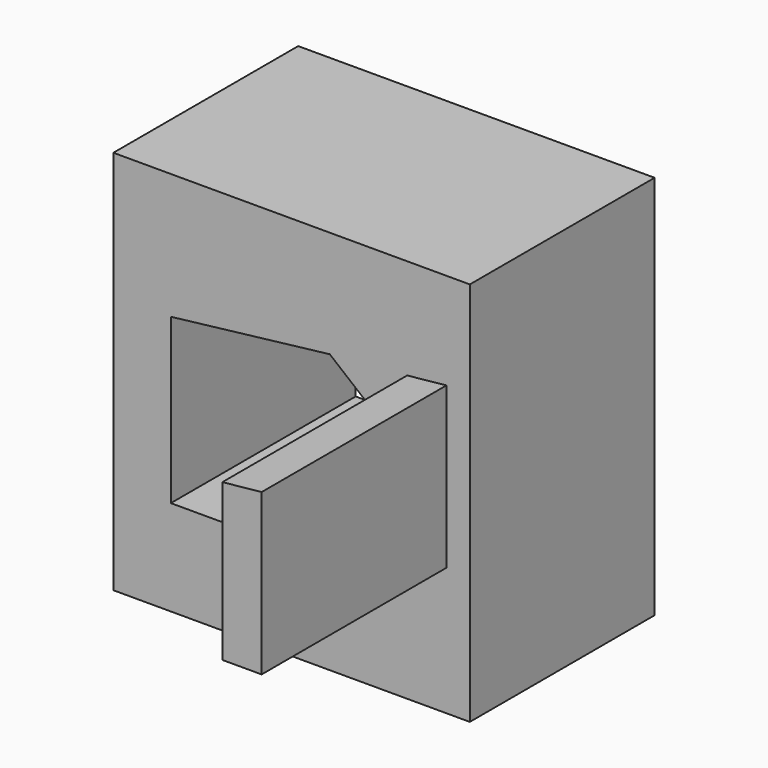
from build123d import *

# Parameters (mm, degrees)
F0_W     = 39.1931459308
F0_H     = 42.3528775573
F1_DEPTH = 25.4
F3_DEPTH = 25.4
F5_DEPTH = 25.4


# Not quite as in the source:
# - ends of sketch curves that miss each other by under 0.0002 mm in the source are joined
# - a feature of the source that left no trace in its solid (it failed there, or was rolled back) is left out


with BuildPart() as f1:
    # F0 (on Front) → F1 (new body)
    with BuildSketch(Plane.XZ):
        with Locations((-19.5965729654, 21.1764387786)):
            Rectangle(F0_W, F0_H)
    extrude(amount=F1_DEPTH)

    # F2 (on face) → F3 (cut)
    with BuildSketch(Plane.XZ.offset(25.4)):
        Polygon((-6.8881497718, 23.612594232), (-15.3977563605, 30.5856615305), (-32.8769646585, 28.529709205), (-32.8769646585, 10.48855111), (-16.7776942253, 10.48855111), (-14.3628085498, 20.764878951), align=None)
        Polygon((-21.8374673277, 17.9171636701), (-14.3628085498, 20.764878951), (-20.9175087512, 15.6267150305), align=None, mode=Mode.SUBTRACT)
        Polygon((-20.9175087512, 15.6267150305), (-14.3628085498, 20.764878951), (-21.8374673277, 17.9171636701), align=None)
    extrude(amount=-F3_DEPTH, mode=Mode.SUBTRACT)

    # F4 (on face) → F5 (join)
    with BuildSketch(Plane.XZ.offset(25.4)):
        Polygon((-6.8881497718, 31.2989987433), (-6.8881497718, 23.612594232), (-6.8881497718, 14.083658345), (-2.5741870049, 14.083658345), (-2.5741870049, 31.7389145494), align=None)
    extrude(amount=F5_DEPTH)


solid = f1.part
